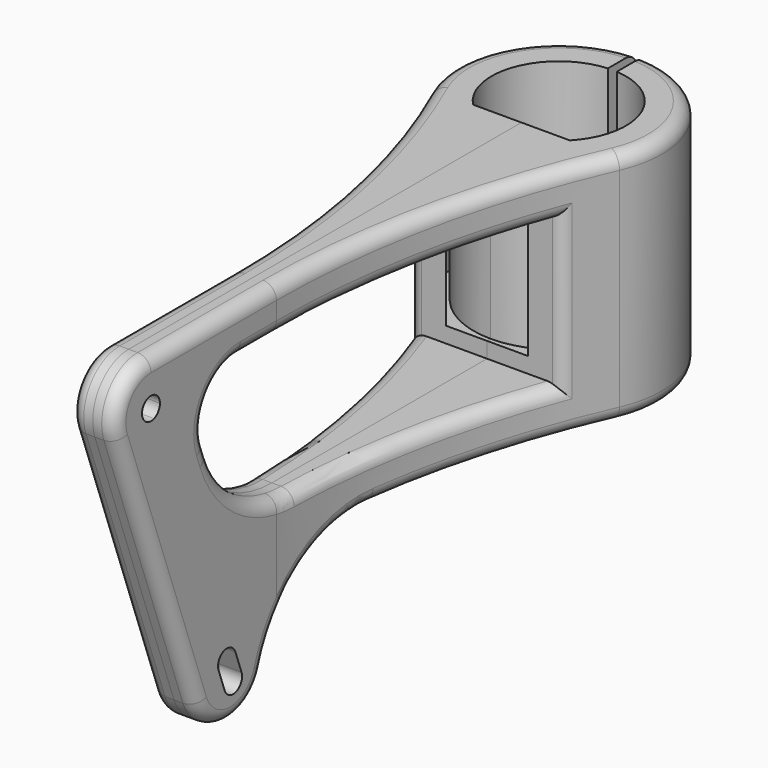
from build123d import *

# Parameters (mm, degrees)
F1_DEPTH = 100
F3_DEPTH = 23.001
F4_W     = 3
F4_H     = 26
F6_R     = 3


# Not quite as in the source:
# - ends of sketch curves that miss each other by under 0.0002 mm in the source are joined


with BuildPart() as f1:
    # F0 (on Top) → F1 (new body)
    with BuildSketch(Plane.XY):
        with BuildLine():
            ThreePointArc((1.0000008821, 14.9666294882), (13.990393338, 5.410073405), (10.8092552935, -10.4))
            Line((10.8092552935, -10.4), (0, -10.4))
            Line((0, -10.4), (0, -170))
            Line((0, -170), (5, -170))
            Line((5, -170), (5, -85))
            ThreePointArc((5, -85), (9.0503612601, -46.3224294433), (21.025698768, -9.3230891509))
            ThreePointArc((21.025698768, -9.3230891509), (19.5480686708, 12.1191175934), (1, 22.9782505862))
            Line((1, 22.9782505862), (1.0000008821, 14.9666294882))
        make_face()
    extrude(amount=-F1_DEPTH)

    # F2 (on Right) → F3 (cut, through all)
    with BuildSketch(Plane.YZ):
        with BuildLine():
            ThreePointArc((-119.1449496417, -12.349231552), (-117.9521198893, -11.4339410909), (-117.5, -10))
            ThreePointArc((-117.5, -10), (-122.0478801107, -8.5660589091), (-119.1449496417, -12.349231552))
        make_face()
        with BuildLine():
            ThreePointArc((-96.4455195618, -67.4058921304), (-97.7382054595, -65.9951730211), (-99.6498014721, -65.9117109368))
            ThreePointArc((-99.6498014721, -65.9117109368), (-101.0605205814, -67.2043968344), (-101.1439826658, -69.115992847))
            Line((-101.1439826658, -69.115992847), (-99.4338819491, -73.814455951))
            ThreePointArc((-99.4338819491, -73.814455951), (-96.2296000389, -75.3086371446), (-94.7354188452, -72.1043552343))
            Line((-94.7354188452, -72.1043552343), (-96.4455195618, -67.4058921304))
        make_face()
        with BuildLine():
            Line((-104.4736684157, -23.4202014333), (-103.516316726, -26.0505035831))
            ThreePointArc((-103.516316726, -26.0505035831), (-94.3634121151, -37.9788011072), (-80.0240012063, -42.5))
            Line((-80.0240012063, -42.5), (-20, -42.5))
            Line((-20, -42.5), (-20, -10))
            Line((-20, -10), (-95.0767422078, -10))
            ThreePointArc((-95.0767422078, -10), (-103.2682626507, -14.2642356365), (-104.4736684157, -23.4202014333))
        make_face()
        with BuildLine():
            Line((-170, 0), (-170, -100))
            Line((-170, -100), (22.9782505862, -100))
            Line((22.9782505862, -100), (22.9782505862, -52.5))
            Line((22.9782505862, -52.5), (-59.7476591937, -52.5))
            ThreePointArc((-59.7476591937, -52.5), (-77.5307820341, -58.3388629812), (-88.391690365, -73.5826305305))
            ThreePointArc((-88.391690365, -73.5826305305), (-97.7034265691, -80.6073823765), (-107.3366269634, -74.0303754739))
            Line((-107.3366269634, -74.0303754739), (-129.3969262079, -13.4202014333))
            ThreePointArc((-129.3969262079, -13.4202014333), (-128.1915204429, -4.2642356365), (-120, 0))
            Line((-120, 0), (-170, 0))
        make_face()
    extrude(amount=F3_DEPTH, mode=Mode.SUBTRACT)

    # F4 (on Right) → F5 (revolve, cut)
    with BuildSketch(Plane.YZ):
        with Locations((-20.5, -26)):
            Rectangle(F4_W, F4_H)
    revolve(axis=Axis((0, 0, -112.1668060077), (0, 0, -1)), mode=Mode.SUBTRACT)

    # F6
    f6_edges = [f1.edges().sort_by_distance(p)[0] for p in [
        (5, -118.366777, -43.725288),
        (8.399785, -49.533347, -42.5),
        (16.680686, -20, -26.25),
    ]]
    fillet(f6_edges, radius=F6_R)


with BuildPart() as f7_1:
    # F7: instance of F1
    add(f1.part.mirror(Plane.YZ))


solid = Compound([f1.part, f7_1.part])
